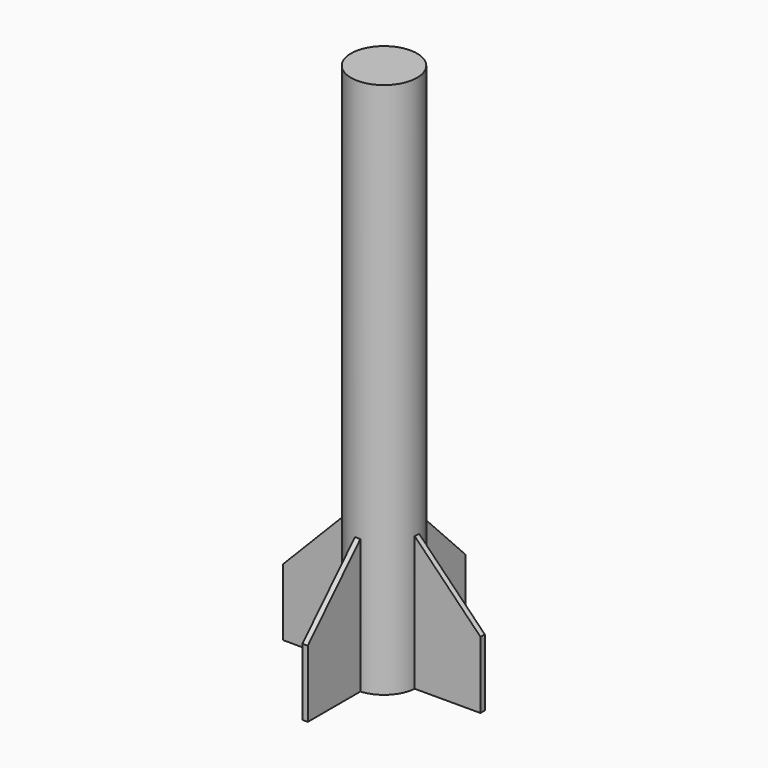
from build123d import *

# Parameters (mm, degrees)
F3_DEPTH = 1
F4_COUNT = 4


with BuildPart() as f1:
    # F0 (on Front) → F1 (revolve)
    with BuildSketch(Plane.XZ):
        Polygon((-12.3, 0), (-11.5, 0), (-11.5, 198), (0, 198), (0, 200), (-12.3, 200), align=None)
    revolve(axis=Axis((0, 0, 95.4308453947), (0, 0, 1)))


with BuildPart() as f3:
    # F2 (on Right) → F3 (new body, symmetric)
    with BuildSketch(Plane.YZ):
        Polygon((-36.7370644584, 0), (-11.7370644584, 0), (-12.2474459931, 50.0576272607), (-36.7370644584, 25), align=None)
    extrude(amount=F3_DEPTH, both=True)


with BuildPart() as f4_1:
    # F4: instance of F3
    add(f3.part.rotate(Axis((0, 0, 200), (0, 0, -1)), 1 * 360 / F4_COUNT))


with BuildPart() as f4_2:
    # F4: instance of F3
    add(f3.part.rotate(Axis((0, 0, 200), (0, 0, -1)), 2 * 360 / F4_COUNT))


with BuildPart() as f4_3:
    # F4: instance of F3
    add(f3.part.rotate(Axis((0, 0, 200), (0, 0, -1)), 3 * 360 / F4_COUNT))


solid = Compound([f1.part, f3.part, f4_1.part, f4_2.part, f4_3.part])
